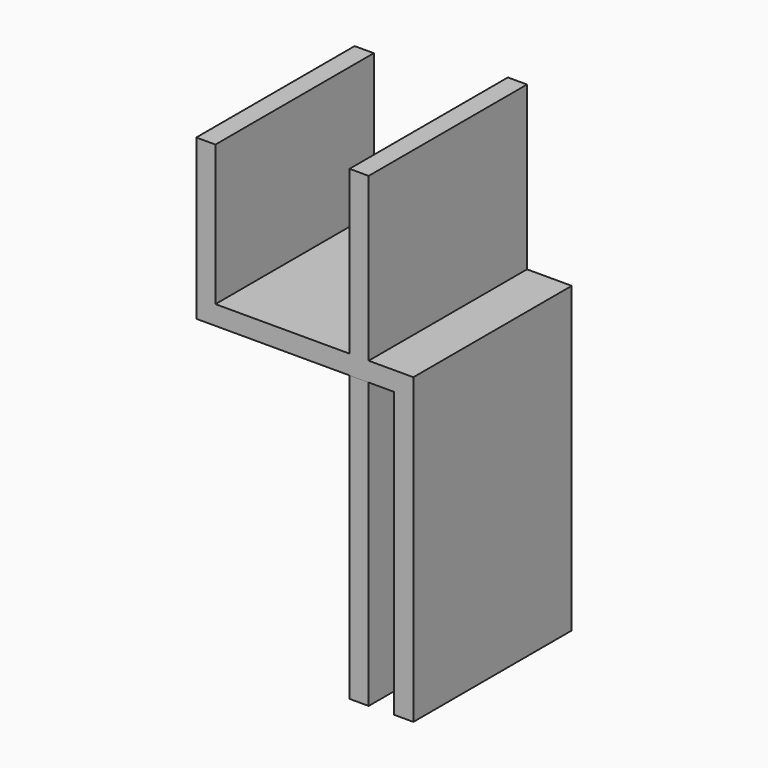
from build123d import *

# Parameters (mm, degrees)
F0_W      = 4
F0_H      = 31
F1_DEPTH  = 3
F2_W      = 31
F2_H      = 47.5263299036
F3_DEPTH  = 3
F4_W      = 31
F4_H      = 44.6022309436
F5_DEPTH  = 3
F6_W      = 24
F6_H      = 31
F7_DEPTH  = 3
F8_W      = 3
F8_H      = 31
F9_DEPTH  = 25
F10_W     = 31
F10_H     = 28.4836739302
F11_DEPTH = 3


with BuildPart() as f1:
    # F0 (on Top) → F1 (new body)
    with BuildSketch(Plane.XY):
        with Locations((-12.1510221595, -3.5323435441)):
            Rectangle(F0_W, F0_H)
    extrude(amount=F1_DEPTH)

    # F2 (on face) → F3 (join)
    with BuildSketch(Plane.YZ.offset(-10.1510221595)):
        with Locations((-3.5323435441, -20.7631649518)):
            Rectangle(F2_W, F2_H)
    extrude(amount=F3_DEPTH)

    # F6 (on face) → F7 (join)
    with BuildSketch(Plane.XY.offset(3)):
        with Locations((-26.1510221595, -3.5323435441)):
            Rectangle(F6_W, F6_H)
    extrude(amount=-F7_DEPTH)

    # F8 (on face) → F9 (join)
    with BuildSketch(Plane(origin=(0, 0, 0), x_dir=(1, 0, 0), z_dir=(0, 0, -1))):
        with Locations((-39.6510221595, 3.5323435441)):
            Rectangle(F8_W, F8_H)
    extrude(amount=-F9_DEPTH)

    # F10 (on face) → F11 (join)
    with BuildSketch(Plane(origin=(-17.1510221595, 0, 0), x_dir=(0, -1, 0), z_dir=(-1, 0, 0))):
        with Locations((3.5323435441, 14.2418369651)):
            Rectangle(F10_W, F10_H)
    extrude(amount=-F11_DEPTH)


with BuildPart() as f5:
    # F4 (on face) → F5 (new body)
    with BuildSketch(Plane(origin=(-14.1510221595, 0, 0), x_dir=(0, -1, 0), z_dir=(-1, 0, 0))):
        with Locations((3.5323435441, -22.3011154718)):
            Rectangle(F4_W, F4_H)
    extrude(amount=F5_DEPTH)


solid = Compound([f1.part, f5.part])
